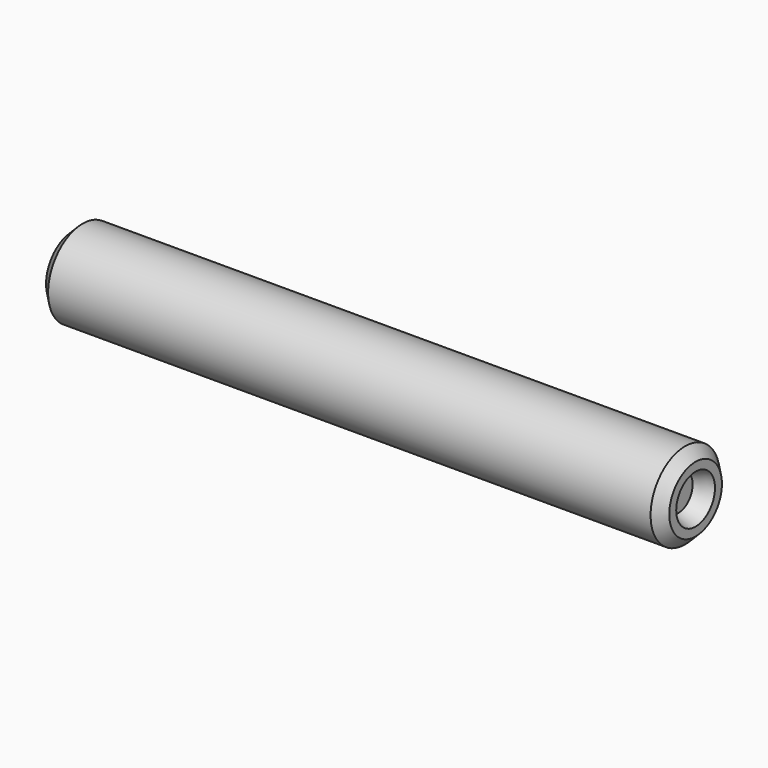
from build123d import *

# Parameters (mm, degrees)
F0_R     = 1.25
F1_DEPTH = 9
F2_SIZE  = 0.3
F3_R     = 0.7
F4_DEPTH = 0.5
F4_TAPER = 20


# Not quite as in the source:
# - a pattern or mirror of a feature is missing from the dataset's text; its kind, count and spacing are read off the source's solid


with BuildPart() as f1:
    # F0 (on Right) → F1 (new body, symmetric)
    with BuildSketch(Plane.YZ):
        Circle(F0_R)
    extrude(amount=F1_DEPTH, both=True)

    # F2
    f2_edges = [f1.edges().sort_by_distance(p)[0] for p in [
        (-9, -1.25, 0),
        (9, -1.25, 0),
    ]]
    chamfer(f2_edges, length=F2_SIZE)

    # F3 (on face) → F4 (cut)
    with BuildSketch(Plane(origin=(-9, 0, 0), x_dir=(0, -1, 0), z_dir=(-1, 0, 0))):
        Circle(F3_R)
    f4 = extrude(amount=-F4_DEPTH, taper=F4_TAPER, mode=Mode.SUBTRACT)

    # F4_copies: F4 across plane
    add(f4.mirror(Plane(origin=(0, 0, 0), x_dir=(0, 0, 1), z_dir=(1, 0, 0))), mode=Mode.SUBTRACT)


solid = f1.part
